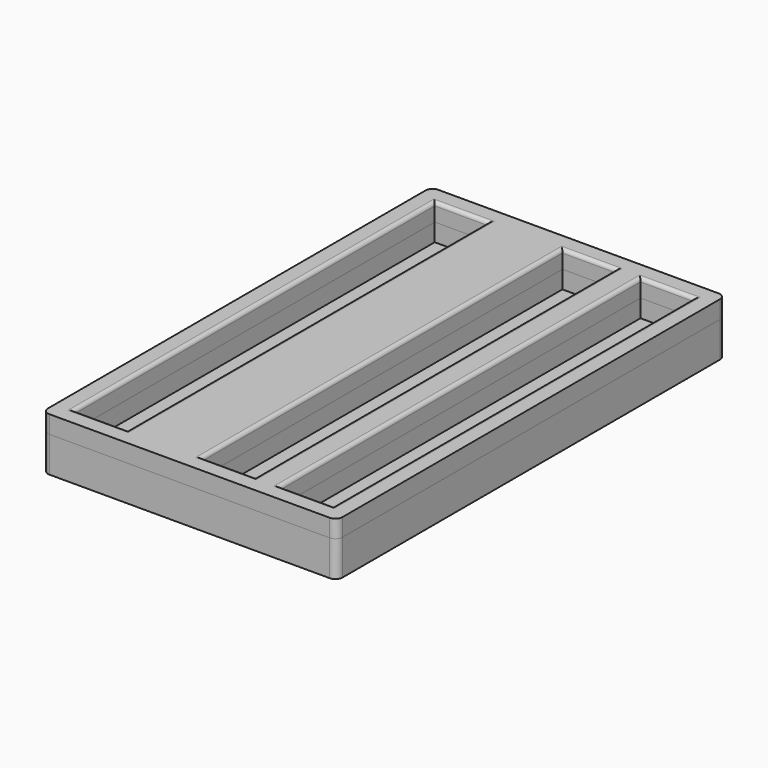
from build123d import *

# Parameters (mm, degrees)
F1_W     = 83
F1_H     = 137
F2_DEPTH = 5
F0_W     = 15
F0_H     = 127
F3_DEPTH = 25
F4_R     = 2
F5_DEPTH = 5
F6_R     = 1


with BuildPart() as f2:
    # F1 (on Top) → F2 (new body, symmetric)
    with BuildSketch(Plane.XY):
        Rectangle(F1_W, F1_H)
    extrude(amount=F2_DEPTH, both=True)

    # F0 (on Top) → F3 (cut)
    with BuildSketch(Plane.XY):
        with Locations((-29, 0)):
            Rectangle(F0_W, F0_H)
        with Locations((29, 0)):
            Rectangle(F0_W, F0_H)
        with Locations((7, 0)):
            Rectangle(F0_W, F0_H)
    extrude(amount=F3_DEPTH, mode=Mode.SUBTRACT)

    # F4
    f4_edges = [f2.edges().sort_by_distance(p)[0] for p in [
        (-41.5, -68.5, 0),
        (41.5, -68.5, 0),
        (41.5, 68.5, 0),
        (-41.5, 68.5, 0),
    ]]
    fillet(f4_edges, radius=F4_R)

    # F5 (add): a face of the model
    f5_faces = [f2.faces().sort_by_distance(p)[0] for p in [
        (-2.3591054268, 0, 5),
    ]]
    extrude(f5_faces, amount=F5_DEPTH)

    # F6
    f6_edges = [f2.edges().sort_by_distance(p)[0] for p in [
        (-21.5, 0, 10),
        (-29, 63.5, 10),
        (-36.5, 0, 10),
        (-29, -63.5, 10),
        (-0.5, 0, 10),
        (14.5, 0, 10),
        (7, 63.5, 10),
        (7, -63.5, 10),
        (29, 63.5, 10),
        (21.5, 0, 10),
        (36.5, 0, 10),
        (29, -63.5, 10),
    ]]
    fillet(f6_edges, radius=F6_R)


solid = f2.part
